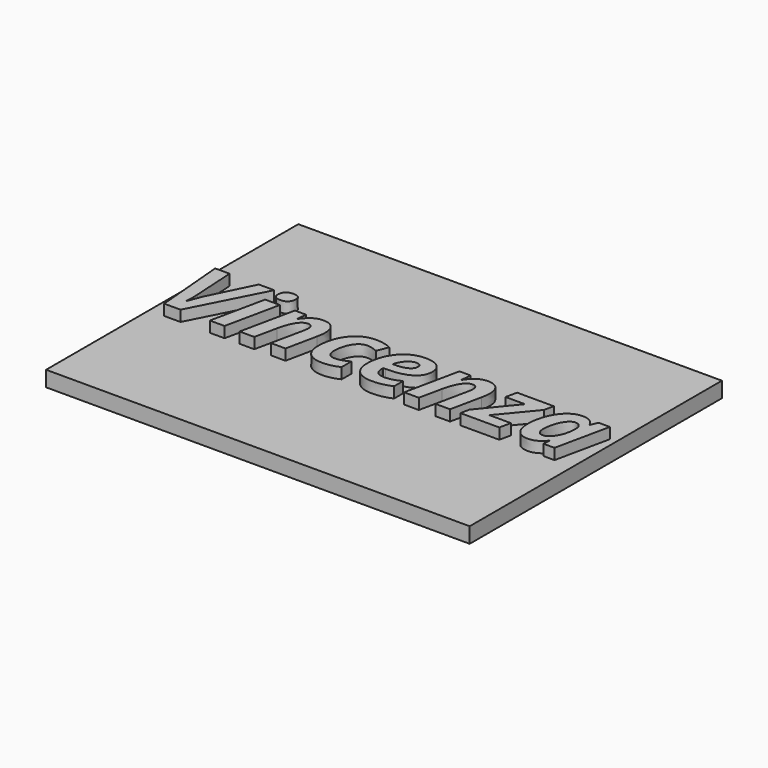
from build123d import *

# Parameters (mm, degrees)
F0_W         = 136.8114054203
F0_H         = 101.8205136061
F1_DEPTH     = 5
F2_TEXT_SIZE = 32.3264045887
F3_DEPTH     = 3.5


# Not quite as in the source:
# - Text() gives the source's letters only with a copy of the font that has no kerning and outlines rounded to 1/6400 em; it was checked with that copy


with BuildPart() as f1:
    # F0 (on Top) → F1 (new body)
    with BuildSketch(Plane.XY):
        Rectangle(F0_W, F0_H)
    extrude(amount=F1_DEPTH)

    # F2 (on face) → F3 (join)
    with BuildSketch(Plane.XY.offset(5)):
        with Locations((-68.4057027102, -9.3621770203)):
            Text('Vincenza', F2_TEXT_SIZE, font='Open Sans', font_style=FontStyle.BOLDITALIC, text_align=(TextAlign.LEFT, TextAlign.BOTTOM))
    extrude(amount=F3_DEPTH)


solid = f1.part
